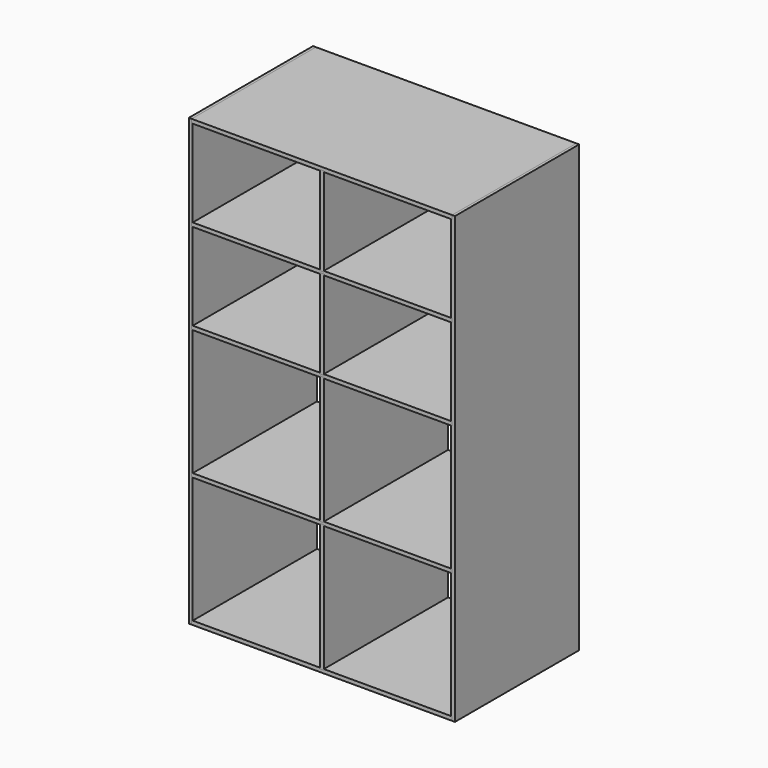
from build123d import *

# Parameters (mm, degrees)
F2_DEPTH = 598
F3_DEPTH = 598
F4_DEPTH = 598
F5_DEPTH = 598
F6_DEPTH = 598
F7_DEPTH = 598
F8_DEPTH = 598


# Not quite as in the source:
# - a feature names something its author has since deleted; it is built from what else it names


with BuildPart() as f2:
    # F1 (on Front) → F2 (new body)
    with BuildSketch(Plane.XZ):
        Polygon((-501.5, 842.5), (-501.5, 857.5), (-512.5, 857.5), (-512.5, -857.5), (-501.5, -857.5), (-501.5, -842.5), (-497.5, -842.5), (-497.5, -357.5), (-501.5, -357.5), (-501.5, -342.5), (-497.5, -342.5), (-497.5, 142.5), (-501.5, 142.5), (-501.5, 157.5), (-497.5, 157.5), (-497.5, 492.5), (-501.5, 492.5), (-501.5, 507.5), (-497.5, 507.5), (-497.5, 842.5), align=None)
    extrude(amount=-F2_DEPTH)


with BuildPart() as f3:
    # F1 (on Front) → F3 (new body)
    with BuildSketch(Plane.XZ):
        Polygon((501.5, 842.5), (497.5, 842.5), (497.5, 507.5), (501.5, 507.5), (501.5, 492.5), (497.5, 492.5), (497.5, 157.5), (501.5, 157.5), (501.5, 142.5), (497.5, 142.5), (497.5, -342.5), (501.5, -342.5), (501.5, -357.5), (497.5, -357.5), (497.5, -842.5), (501.5, -842.5), (501.5, -857.5), (512.5, -857.5), (512.5, 857.5), (501.5, 857.5), align=None)
    extrude(amount=-F3_DEPTH)


with BuildPart() as f4:
    # F1 (on Front) → F4 (new body)
    with BuildSketch(Plane.XZ):
        Polygon((7.5, 842.5), (497.5, 842.5), (501.5, 842.5), (501.5, 857.5), (-501.5, 857.5), (-501.5, 842.5), (-497.5, 842.5), (-7.5, 842.5), (-7.5, 846.5), (7.5, 846.5), align=None)
    extrude(amount=-F4_DEPTH)


with BuildPart() as f4b:
    # F1 (on Front) → F4, piece 2 (new body)
    with BuildSketch(Plane.XZ):
        Polygon((-501.5, -857.5), (501.5, -857.5), (501.5, -842.5), (497.5, -842.5), (7.5, -842.5), (7.5, -846.5), (-7.5, -846.5), (-7.5, -842.5), (-497.5, -842.5), (-501.5, -842.5), align=None)
    extrude(amount=-F4_DEPTH)


with BuildPart() as f5:
    # F1 (on Front) → F5 (new body)
    with BuildSketch(Plane.XZ):
        Polygon((7.5, -357.5), (497.5, -357.5), (501.5, -357.5), (501.5, -342.5), (497.5, -342.5), (7.5, -342.5), (7.5, -346.5), (-7.5, -346.5), (-7.5, -342.5), (-497.5, -342.5), (-501.5, -342.5), (-501.5, -357.5), (-497.5, -357.5), (-7.5, -357.5), (-7.5, -353.5), (7.5, -353.5), align=None)
    extrude(amount=-F5_DEPTH)


with BuildPart() as f6:
    # F1 (on Front) → F6 (new body)
    with BuildSketch(Plane.XZ):
        Polygon((7.5, 507.5), (7.5, 842.5), (7.5, 846.5), (-7.5, 846.5), (-7.5, 842.5), (-7.5, 507.5), (-7.5, 503.5), (7.5, 503.5), align=None)
    extrude(amount=-F6_DEPTH)


with BuildPart() as f6b:
    # F1 (on Front) → F6, piece 2 (new body)
    with BuildSketch(Plane.XZ):
        Polygon((7.5, 157.5), (7.5, 492.5), (7.5, 496.5), (-7.5, 496.5), (-7.5, 492.5), (-7.5, 157.5), (-7.5, 153.5), (7.5, 153.5), align=None)
    extrude(amount=-F6_DEPTH)


with BuildPart() as f7:
    # F1 (on Front) → F7 (new body)
    with BuildSketch(Plane.XZ):
        Polygon((7.5, -846.5), (7.5, -842.5), (7.5, -357.5), (7.5, -353.5), (-7.5, -353.5), (-7.5, -357.5), (-7.5, -842.5), (-7.5, -846.5), align=None)
    extrude(amount=-F7_DEPTH)


with BuildPart() as f7b:
    # F1 (on Front) → F7, piece 2 (new body)
    with BuildSketch(Plane.XZ):
        Polygon((7.5, -342.5), (7.5, 142.5), (7.5, 146.5), (-7.5, 146.5), (-7.5, 142.5), (-7.5, -342.5), (-7.5, -346.5), (7.5, -346.5), align=None)
    extrude(amount=-F7_DEPTH)


with BuildPart() as f8:
    # F1 (on Front) → F8 (new body)
    with BuildSketch(Plane.XZ):
        Polygon((501.5, 507.5), (497.5, 507.5), (7.5, 507.5), (7.5, 503.5), (-7.5, 503.5), (-7.5, 507.5), (-497.5, 507.5), (-501.5, 507.5), (-501.5, 492.5), (-497.5, 492.5), (-7.5, 492.5), (-7.5, 496.5), (7.5, 496.5), (7.5, 492.5), (497.5, 492.5), (501.5, 492.5), align=None)
    extrude(amount=-F8_DEPTH)


with BuildPart() as f8b:
    # F1 (on Front) → F8, piece 2 (new body)
    with BuildSketch(Plane.XZ):
        Polygon((501.5, 157.5), (497.5, 157.5), (7.5, 157.5), (7.5, 153.5), (-7.5, 153.5), (-7.5, 157.5), (-497.5, 157.5), (-501.5, 157.5), (-501.5, 142.5), (-497.5, 142.5), (-7.5, 142.5), (-7.5, 146.5), (7.5, 146.5), (7.5, 142.5), (497.5, 142.5), (501.5, 142.5), align=None)
    extrude(amount=-F8_DEPTH)


solid = Compound([f2.part, f3.part, f4.part, f4b.part, f5.part, f6.part, f6b.part, f7.part, f7b.part, f8.part, f8b.part])
